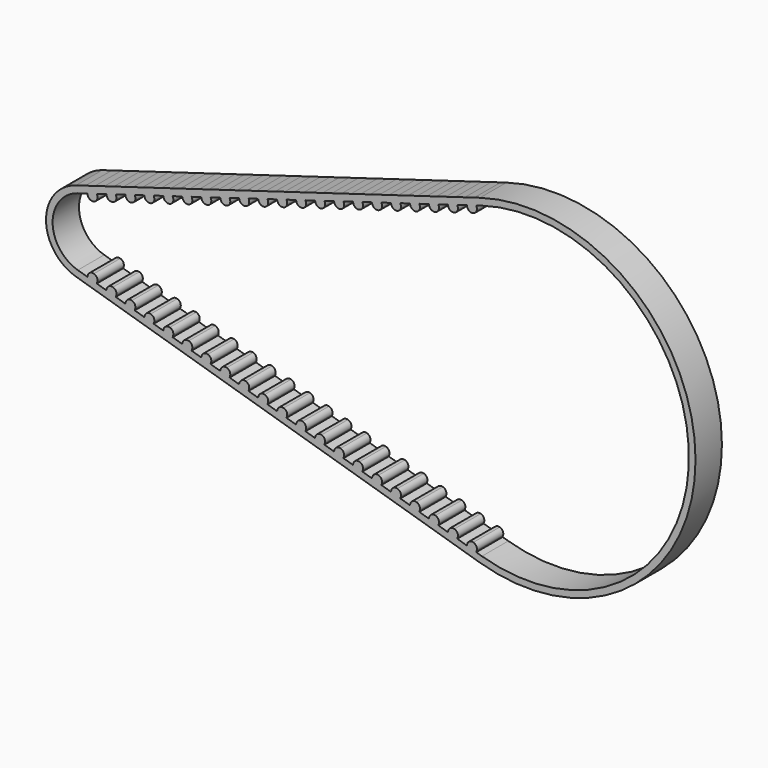
from build123d import *

# Parameters (mm, degrees)
F1_DEPTH = 10
F2_T     = -2
F3_W     = 3
F3_H     = 10
F4_DEPTH = 4
F5_R     = 1.5
F6_R     = 1.49999
F7_W     = 3
F7_H     = 10
F8_DEPTH = 4
F9_R     = 1.49999


# Not quite as in the source:
# - a fillet or chamfer is up to 0.001 mm smaller than in the source, because OpenCascade refuses the exact size


with BuildPart() as f1:
    # F0 (on Front) → F1 (new body)
    with BuildSketch(Plane.XZ):
        with BuildLine():
            Line((43.0367631963, 48.682394253), (-79.427522518, 12.1705985632))
            ThreePointArc((-79.427522518, 12.1705985632), (-88.4989510894, 0), (-79.427522518, -12.1705985632))
            Line((-79.427522518, -12.1705985632), (43.0367631963, -48.682394253))
            ThreePointArc((43.0367631963, -48.682394253), (108.3510489106, 0), (43.0367631963, 48.682394253))
        make_face()
    extrude(amount=F1_DEPTH)

    # F2
    f2_openings = [f1.faces().sort_by_distance(p)[0] for p in [
        (25.608831, -10, 0),
        (25.608831, 0, 0),
    ]]
    offset(amount=F2_T, openings=f2_openings)

    # F3 (on face) → F4 (join)
    with BuildSketch(Plane(origin=(-9.8162409053, 0, 32.9246729215), x_dir=(0.9583148475, 0, 0.2857142857), z_dir=(-0.2857142857, 0, 0.9583148475))):
        with Locations((-68.1392602539, -5)):
            Rectangle(F3_W, F3_H)
        with Locations((-62.1392602539, -5)):
            Rectangle(F3_W, F3_H)
        with Locations((-56.1392602539, -5)):
            Rectangle(F3_W, F3_H)
        with Locations((-50.1392602539, -5)):
            Rectangle(F3_W, F3_H)
        with Locations((-44.1392602539, -5)):
            Rectangle(F3_W, F3_H)
        with Locations((-38.1392602539, -5)):
            Rectangle(F3_W, F3_H)
        with Locations((-32.1392602539, -5)):
            Rectangle(F3_W, F3_H)
        with Locations((-26.1392602539, -5)):
            Rectangle(F3_W, F3_H)
        with Locations((-20.1392602539, -5)):
            Rectangle(F3_W, F3_H)
        with Locations((-14.1392602539, -5)):
            Rectangle(F3_W, F3_H)
        with Locations((-8.1392602539, -5)):
            Rectangle(F3_W, F3_H)
        with Locations((-2.1392602539, -5)):
            Rectangle(F3_W, F3_H)
        with Locations((3.8607397461, -5)):
            Rectangle(F3_W, F3_H)
        with Locations((9.8607397461, -5)):
            Rectangle(F3_W, F3_H)
        with Locations((15.8607397461, -5)):
            Rectangle(F3_W, F3_H)
        with Locations((21.8607397461, -5)):
            Rectangle(F3_W, F3_H)
        with Locations((27.8607397461, -5)):
            Rectangle(F3_W, F3_H)
        with Locations((33.8607397461, -5)):
            Rectangle(F3_W, F3_H)
        with Locations((39.8607397461, -5)):
            Rectangle(F3_W, F3_H)
        with Locations((45.8607397461, -5)):
            Rectangle(F3_W, F3_H)
        with Locations((51.8607397461, -5)):
            Rectangle(F3_W, F3_H)
    extrude(amount=-F4_DEPTH)

    # F5
    f5_edges = [f1.edges().sort_by_distance(p)[0] for p in [
        (-75.409721, -5, 9.194482),
    ]]
    fillet(f5_edges, radius=F5_R)

    # F6 (radius 1.5 in the source; OpenCascade refuses exactly that, so slightly less here)
    f6_edges = [f1.edges().sort_by_distance(p)[0] for p in [
        (-72.534776, -5, 10.051625),
        (-69.659832, -5, 10.908768),
        (-66.784887, -5, 11.765911),
        (-63.909943, -5, 12.623053),
        (-61.034998, -5, 13.480196),
        (-58.160054, -5, 14.337339),
        (-55.285109, -5, 15.194482),
        (-52.410164, -5, 16.051625),
        (-49.53522, -5, 16.908768),
        (-46.660275, -5, 17.765911),
        (-43.785331, -5, 18.623053),
        (-40.910386, -5, 19.480196),
        (-38.035442, -5, 20.337339),
        (-35.160497, -5, 21.194482),
        (-32.285553, -5, 22.051625),
        (-29.410608, -5, 22.908768),
        (-26.535664, -5, 23.765911),
        (-23.660719, -5, 24.623053),
        (-20.785775, -5, 25.480196),
        (-17.91083, -5, 26.337339),
        (-15.035885, -5, 27.194482),
        (-12.160941, -5, 28.051625),
        (-9.285996, -5, 28.908768),
        (-6.411052, -5, 29.765911),
        (-3.536107, -5, 30.623053),
        (-0.661163, -5, 31.480196),
        (2.213782, -5, 32.337339),
        (5.088726, -5, 33.194482),
        (7.963671, -5, 34.051625),
        (10.838615, -5, 34.908768),
        (13.71356, -5, 35.765911),
        (16.588505, -5, 36.623053),
        (19.463449, -5, 37.480196),
        (22.338394, -5, 38.337339),
        (25.213338, -5, 39.194482),
        (28.088283, -5, 40.051625),
        (30.963227, -5, 40.908768),
        (33.838172, -5, 41.765911),
        (36.713116, -5, 42.623053),
        (39.588061, -5, 43.480196),
        (42.463005, -5, 44.337339),
    ]]
    fillet(f6_edges, radius=F6_R)

    # F7 (on face) → F8 (join)
    with BuildSketch(Plane(origin=(-9.8162409053, 0, -32.9246729215), x_dir=(0.9583148475, 0, -0.2857142857), z_dir=(-0.2857142857, 0, -0.9583148475))):
        with Locations((-68.1392602539, 5)):
            Rectangle(F7_W, F7_H)
        with Locations((-62.1392602539, 5)):
            Rectangle(F7_W, F7_H)
        with Locations((-56.1392602539, 5)):
            Rectangle(F7_W, F7_H)
        with Locations((-50.1392602539, 5)):
            Rectangle(F7_W, F7_H)
        with Locations((-44.1392602539, 5)):
            Rectangle(F7_W, F7_H)
        with Locations((-38.1392602539, 5)):
            Rectangle(F7_W, F7_H)
        with Locations((-32.1392602539, 5)):
            Rectangle(F7_W, F7_H)
        with Locations((-26.1392602539, 5)):
            Rectangle(F7_W, F7_H)
        with Locations((-20.1392602539, 5)):
            Rectangle(F7_W, F7_H)
        with Locations((-14.1392602539, 5)):
            Rectangle(F7_W, F7_H)
        with Locations((-8.1392602539, 5)):
            Rectangle(F7_W, F7_H)
        with Locations((-2.1392602539, 5)):
            Rectangle(F7_W, F7_H)
        with Locations((3.8607397461, 5)):
            Rectangle(F7_W, F7_H)
        with Locations((9.8607397461, 5)):
            Rectangle(F7_W, F7_H)
        with Locations((15.8607397461, 5)):
            Rectangle(F7_W, F7_H)
        with Locations((21.8607397461, 5)):
            Rectangle(F7_W, F7_H)
        with Locations((27.8607397461, 5)):
            Rectangle(F7_W, F7_H)
        with Locations((33.8607397461, 5)):
            Rectangle(F7_W, F7_H)
        with Locations((39.8607397461, 5)):
            Rectangle(F7_W, F7_H)
        with Locations((45.8607397461, 5)):
            Rectangle(F7_W, F7_H)
        with Locations((51.8607397461, 5)):
            Rectangle(F7_W, F7_H)
    extrude(amount=-F8_DEPTH)

    # F9 (radius 1.5 in the source; OpenCascade refuses exactly that, so slightly less here)
    f9_edges = [f1.edges().sort_by_distance(p)[0] for p in [
        (-75.409721, -5, -9.194482),
        (-72.534776, -5, -10.051625),
        (-69.659832, -5, -10.908768),
        (-66.784887, -5, -11.765911),
        (-63.909943, -5, -12.623053),
        (-58.160054, -5, -14.337339),
        (-61.034998, -5, -13.480196),
        (-55.285109, -5, -15.194482),
        (-52.410164, -5, -16.051625),
        (-49.53522, -5, -16.908768),
        (-46.660275, -5, -17.765911),
        (-43.785331, -5, -18.623053),
        (-40.910386, -5, -19.480196),
        (-38.035442, -5, -20.337339),
        (-35.160497, -5, -21.194482),
        (-32.285553, -5, -22.051625),
        (-29.410608, -5, -22.908768),
        (-26.535664, -5, -23.765911),
        (-23.660719, -5, -24.623053),
        (-20.785775, -5, -25.480196),
        (-17.91083, -5, -26.337339),
        (-15.035885, -5, -27.194482),
        (-12.160941, -5, -28.051625),
        (-9.285996, -5, -28.908768),
        (-6.411052, -5, -29.765911),
        (-3.536107, -5, -30.623053),
        (-0.661163, -5, -31.480196),
        (2.213782, -5, -32.337339),
        (5.088726, -5, -33.194482),
        (7.963671, -5, -34.051625),
        (10.838615, -5, -34.908768),
        (13.71356, -5, -35.765911),
        (16.588505, -5, -36.623053),
        (19.463449, -5, -37.480196),
        (22.338394, -5, -38.337339),
        (25.213338, -5, -39.194482),
        (28.088283, -5, -40.051625),
        (30.963227, -5, -40.908768),
        (33.838172, -5, -41.765911),
        (36.713116, -5, -42.623053),
        (39.588061, -5, -43.480196),
        (42.463005, -5, -44.337339),
    ]]
    fillet(f9_edges, radius=F9_R)


solid = f1.part
